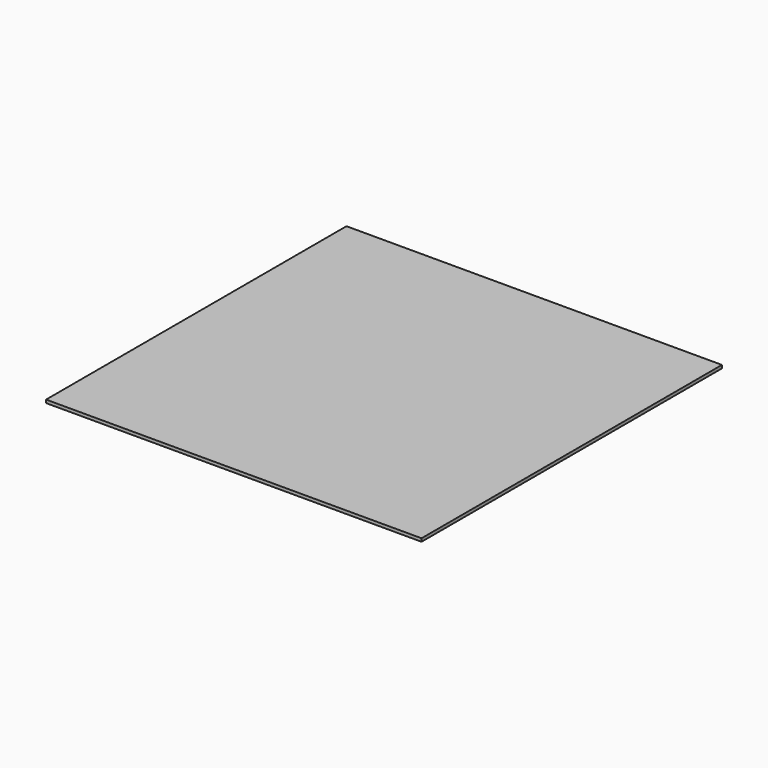
from build123d import *

# Parameters (mm, degrees)
F1_DEPTH = 1


# Not quite as in the source:
# - a feature names something its author has since deleted; it is built from what else it names


with BuildPart() as f1:
    # F0 (on Top) → F1 (new body)
    with BuildSketch(Plane.XY):
        Polygon((-6.35, 56.1535057819), (-127, 56.1535057819), (-127, 11.7035057819), (-127, -64.4964942181), (-6.35, -64.4964942181), (-6.35, 11.7035057819), align=None)
    extrude(amount=F1_DEPTH)


solid = f1.part
